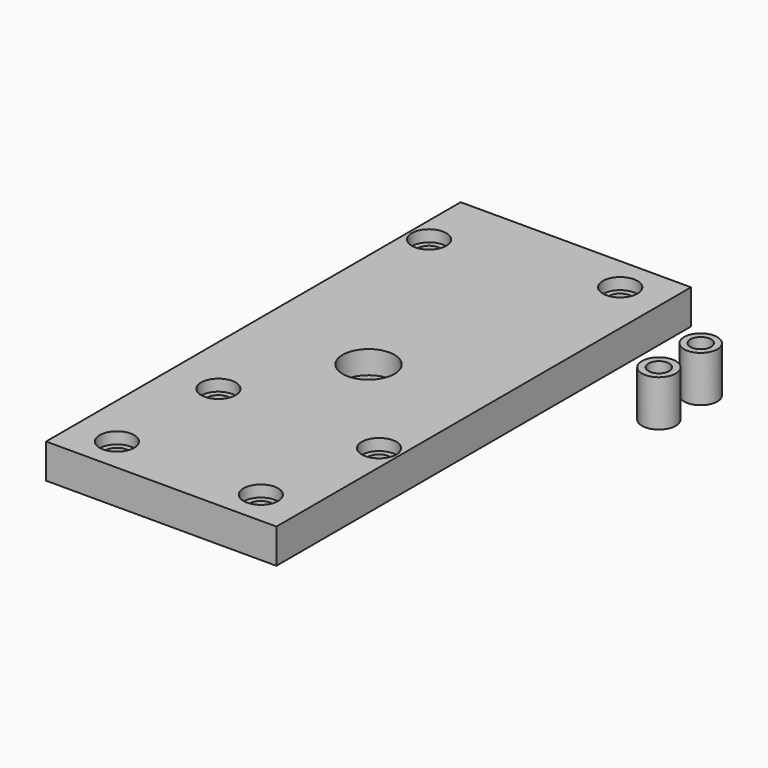
from build123d import *

# Parameters (mm, degrees)
F2_W                 = 40
F2_H                 = 90
F2_R                 = 15
F5_DEPTH             = 6
F6_D                 = 5.5
F6_DEPTH             = 30
F6_CBORE_D           = 9
F6_CBORE_DEPTH       = 4
F6_TIP               = 1.6523667023
F7_D                 = 4
F7_DEPTH             = 30
F7_CBORE_D           = 6
F7_CBORE_DEPTH       = 2
F7_TIP               = 1.2017212381
F7_ON_F4_D           = 4
F7_ON_F4_DEPTH       = 30
F7_ON_F4_CBORE_D     = 6
F7_ON_F4_CBORE_DEPTH = 2
F7_ON_F4_TIP         = 1.2017212381
F7_ON_F3_D           = 4
F7_ON_F3_DEPTH       = 30
F7_ON_F3_CBORE_D     = 6
F7_ON_F3_CBORE_DEPTH = 2
F7_ON_F3_TIP         = 1.2017212381
F2_R_2               = 2.88
F8_DEPTH             = 8
F2_R_3               = 2.94
F9_D                 = 3.6
F9_DEPTH             = 30
F9_TIP               = 1.0815491142
F9_2_D               = 3.6
F9_2_DEPTH           = 30
F9_2_TIP             = 1.0815491142


# Not quite as in the source:
# - a feature names something its author has since deleted; it is built from what else it names


with BuildPart() as f5:
    # F2 (on Top) → F5 (new body)
    with BuildSketch(Plane.XY):
        Rectangle(F2_W, F2_H)
        Circle(F2_R, mode=Mode.SUBTRACT)
        Circle(F2_R)
    extrude(amount=-F5_DEPTH)

    # F6
    with Locations(Plane.XY):
        with Locations((0, 0)):
            CounterBoreHole(F6_D / 2, F6_CBORE_D / 2, F6_CBORE_DEPTH, depth=F6_DEPTH)
            with Locations((0, 0, -(F6_DEPTH + F6_TIP / 2))):  # 118° drill point
                Cone(0, F6_D / 2, F6_TIP, mode=Mode.SUBTRACT)

    # F7
    with Locations(Plane.XY):
        with Locations((12.5, 39), (-16.5140936151, 33.7748509184), (-11.4140936151, -18.3251490816)):
            CounterBoreHole(F7_D / 2, F7_CBORE_D / 2, F7_CBORE_DEPTH, depth=F7_DEPTH)
            with Locations((0, 0, -(F7_DEPTH + F7_TIP / 2))):  # 118° drill point
                Cone(0, F7_D / 2, F7_TIP, mode=Mode.SUBTRACT)

    # F7 on F4
    with Locations(Plane.XY):
        with Locations((16.4859063849, -18.3251490816)):
            CounterBoreHole(F7_ON_F4_D / 2, F7_ON_F4_CBORE_D / 2, F7_ON_F4_CBORE_DEPTH, depth=F7_ON_F4_DEPTH)
            with Locations((0, 0, -(F7_ON_F4_DEPTH + F7_ON_F4_TIP / 2))):  # 118° drill point
                Cone(0, F7_ON_F4_D / 2, F7_ON_F4_TIP, mode=Mode.SUBTRACT)

    # F7 on F3
    with Locations(Plane.XY):
        with Locations((-12.5, -39), (12.5, -39)):
            CounterBoreHole(F7_ON_F3_D / 2, F7_ON_F3_CBORE_D / 2, F7_ON_F3_CBORE_DEPTH, depth=F7_ON_F3_DEPTH)
            with Locations((0, 0, -(F7_ON_F3_DEPTH + F7_ON_F3_TIP / 2))):  # 118° drill point
                Cone(0, F7_ON_F3_D / 2, F7_ON_F3_TIP, mode=Mode.SUBTRACT)


with BuildPart() as f8:
    # F2 (on Top) → F8 (new body)
    with BuildSketch(Plane.XY):
        with Locations((40.8734753728, 21.0164897144)):
            Circle(F2_R_2)
    extrude(amount=F8_DEPTH)

    # F9
    with Locations(Plane(origin=(0, 0, 0), x_dir=(1, 0, 0), z_dir=(0, 0, -1))):
        with Locations((40.8734753728, -11.9312852621), (40.8734753728, -21.0164897144)):
            Hole(F9_D / 2, depth=F9_DEPTH)
            with Locations((0, 0, -(F9_DEPTH + F9_TIP / 2))):  # 118° drill point
                Cone(0, F9_D / 2, F9_TIP, mode=Mode.SUBTRACT)


with BuildPart() as f8b:
    # F2 (on Top) → F8, piece 2 (new body)
    with BuildSketch(Plane.XY):
        with Locations((40.8734753728, 11.9312852621)):
            Circle(F2_R_3)
    extrude(amount=F8_DEPTH)

    # F9#2
    with Locations(Plane(origin=(0, 0, 0), x_dir=(1, 0, 0), z_dir=(0, 0, -1))):
        with Locations((40.8734753728, -11.9312852621), (40.8734753728, -21.0164897144)):
            Hole(F9_2_D / 2, depth=F9_2_DEPTH)
            with Locations((0, 0, -(F9_2_DEPTH + F9_2_TIP / 2))):  # 118° drill point
                Cone(0, F9_2_D / 2, F9_2_TIP, mode=Mode.SUBTRACT)


solid = Compound([f5.part, f8.part, f8b.part])
